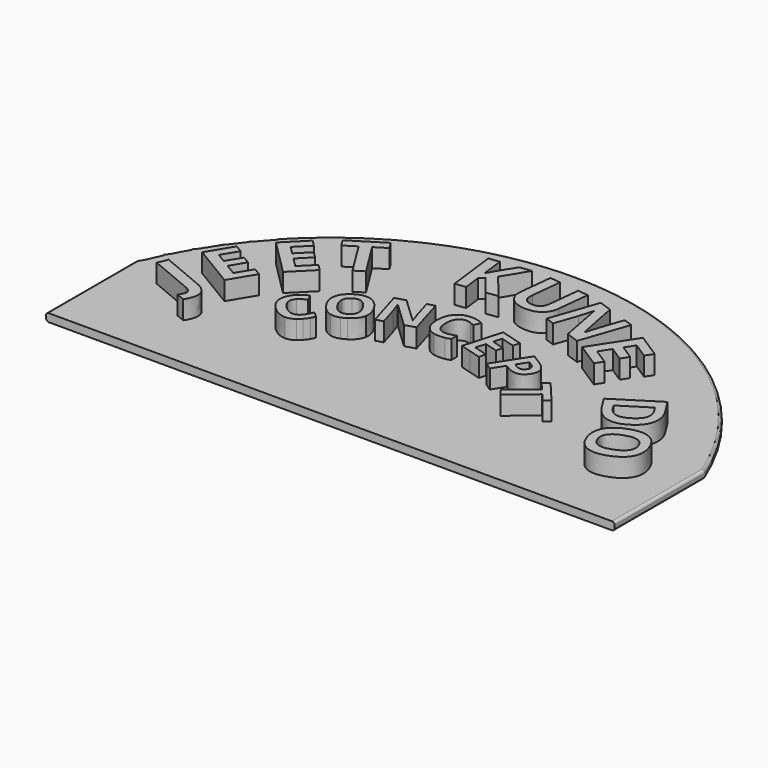
from build123d import *

# Parameters (mm, degrees)
F0_TEXT_SIZE   = 26.3888888889
F0_TEXT_SIZE_2 = 20.8333333333
F1_DEPTH       = 10
F2_W           = 106.8937070169
F2_H           = 42.4115008008
F3_DEPTH       = 3
F4_R           = 1
F5_R           = 1


# Not quite as in the source:
# - Text() gives the source's letters only with a copy of the font that has no kerning and outlines rounded to 1/6400 em; it was checked with that copy


with BuildPart() as f1:
    # F0 (on Top) → F1 (new body)
    with BuildSketch(Plane.XY):
        with BuildLine():
            add(Edge.make_bspline(
                [(-38.4091225358, 32.0256214873), (-39.979942422, 30.889467014), (-41.7688680067, 30.899920348)],
                knots=[0.3156073203, 0.3156073203, 0.3156073203, 1, 1, 1], degree=2))
            Line((-38.4091225358, 32.0256214873), (-35.6095221105, 35.256532611))
            add(Edge.make_bspline(
                [(-34.8738305014, 36.8883343337), (-35.1570391266, 36.0542519462), (-35.6095221105, 35.256532611)],
                knots=[0, 0, 0, 0.4442187703, 0.4442187703, 0.4442187703], degree=2))
            Line((-34.8738305014, 36.8883343337), (-36.8551148685, 38.6379550595))
            add(Edge.make_bspline(
                [(-38.7797452841, 35.2782195153), (-37.7433320216, 36.4518621022), (-36.8551148685, 38.6379550595)],
                knots=[0, 0, 0, 1, 1, 1], degree=2))
            add(Edge.make_bspline(
                [(-44.9795205124, 35.7719230867), (-41.2511922945, 32.4795333465), (-38.7797452841, 35.2782195153)],
                knots=[0, 0, 0, 1, 1, 1], degree=2))
            add(Edge.make_bspline(
                [(-47.1269150723, 38.9710622999), (-46.77048446, 37.3534767969), (-44.9795205124, 35.7719230867)],
                knots=[0, 0, 0, 1, 1, 1], degree=2))
            add(Edge.make_bspline(
                [(-46.3047218705, 41.9233307448), (-47.4833456845, 40.588647803), (-47.1269150723, 38.9710622999)],
                knots=[0, 0, 0, 1, 1, 1], degree=2))
            add(Edge.make_bspline(
                [(-44.9871563721, 42.9702926502), (-45.7660455386, 42.5333320894), (-46.3047218705, 41.9233307448)],
                knots=[0, 0, 0, 1, 1, 1], degree=2))
            add(Edge.make_bspline(
                [(-43.3568272803, 43.7714605433), (-44.2082672056, 43.407253211), (-44.9871563721, 42.9702926502)],
                knots=[0, 0, 0, 1, 1, 1], degree=2))
            Line((-43.3568272803, 43.7714605433), (-44.6072834562, 46.2306500193))
            add(Edge.make_bspline(
                [(-48.2713662053, 43.6600232387), (-46.8384871626, 45.2826268152), (-44.6072834562, 46.2306500193)],
                knots=[0, 0, 0, 1, 1, 1], degree=2))
            add(Edge.make_bspline(
                [(-50.0289540377, 40.2656887419), (-49.6783887841, 42.0666997267), (-48.2713662053, 43.6600232387)],
                knots=[0, 0, 0, 1, 1, 1], degree=2))
            add(Edge.make_bspline(
                [(-49.630822441, 36.6765743061), (-50.3795192913, 38.4646777572), (-50.0289540377, 40.2656887419)],
                knots=[0, 0, 0, 1, 1, 1], degree=2))
            add(Edge.make_bspline(
                [(-47.1424017561, 33.3521659566), (-48.8821255907, 34.888470855), (-49.630822441, 36.6765743061)],
                knots=[0, 0, 0, 1, 1, 1], degree=2))
            add(Edge.make_bspline(
                [(-41.7688680067, 30.899920348), (-44.3827556733, 30.9151942313), (-47.1424017561, 33.3521659566)],
                knots=[0, 0, 0, 1, 1, 1], degree=2))
        make_face()
        with BuildLine():
            Line((-35.6095221105, 35.256532611), (-38.4091225358, 32.0256214873))
            add(Edge.make_bspline(
                [(-37.0067391286, 33.3173318267), (-37.6847397807, 32.5495585185), (-38.4091225358, 32.0256214873)],
                knots=[0, 0, 0, 0.3156073203, 0.3156073203, 0.3156073203], degree=2))
            add(Edge.make_bspline(
                [(-35.6095221105, 35.256532611), (-36.1756430537, 34.2584716043), (-37.0067391286, 33.3173318267)],
                knots=[0.4442187703, 0.4442187703, 0.4442187703, 1, 1, 1], degree=2))
        make_face()
        Polygon((36.4704009429, 34.3043494452), (37.7874787177, 32.7430366973), (38.5155209345, 31.9028311896), (47.867163069, 39.7916030132), (50.4698346878, 36.7062997345), (52.4752818189, 38.3980362866), (45.2339777183, 46.9821462153), (43.2285305872, 45.2904096631), (45.8333011347, 42.2026182366), align=None)
        Polygon((38.5155209345, 31.9028311896), (37.7874787177, 32.7430366973), (38.5042628772, 31.8933342217), align=None)
        Polygon((14.3201833544, 63.3800999888), (10.2276517863, 49.1077462863), (14.0866278421, 47.9746486807), (18.4532967766, 46.7225265126), (19.1711023907, 49.2258121791), (13.9705264185, 50.7170533424), (15.0274951853, 54.4031414864), (19.8682238429, 53.0150848801), (20.5806459149, 55.4995959041), (15.7399172573, 56.8876525104), (16.639866046, 60.0261469147), (21.8404420181, 58.5349057514), (22.5528640902, 61.0194167754), align=None)
        Polygon((14.0866278421, 47.9746486807), (10.2276517863, 49.1077462863), (10.2206160409, 49.083209726), align=None)
        with BuildLine():
            add(Edge.make_bspline(
                [(-0.9883344196, 50), (-2.852809563, 50.430438258), (-4.0169270833, 51.7643229167)],
                knots=[0.3226952609, 0.3226952609, 0.3226952609, 1, 1, 1], degree=2))
            Line((-0.9883344196, 50), (3.1714734134, 50))
            add(Edge.make_bspline(
                [(5.0358072917, 50.5598958333), (4.1536014918, 50.191001949), (3.1714734134, 50)],
                knots=[0, 0, 0, 0.4822306436, 0.4822306436, 0.4822306436], degree=2))
            Line((5.0358072917, 50.5598958333), (5.0358072917, 53.203125))
            add(Edge.make_bspline(
                [(1.2434895833, 52.421875), (2.8092447917, 52.421875), (5.0358072917, 53.203125)],
                knots=[0, 0, 0, 1, 1, 1], degree=2))
            add(Edge.make_bspline(
                [(-2.490234375, 57.3958333333), (-2.490234375, 52.421875), (1.2434895833, 52.421875)],
                knots=[0, 0, 0, 1, 1, 1], degree=2))
            add(Edge.make_bspline(
                [(-1.513671875, 61.123046875), (-2.490234375, 59.78515625), (-2.490234375, 57.3958333333)],
                knots=[0, 0, 0, 1, 1, 1], degree=2))
            add(Edge.make_bspline(
                [(1.2434895833, 62.4609375), (-0.537109375, 62.4609375), (-1.513671875, 61.123046875)],
                knots=[0, 0, 0, 1, 1, 1], degree=2))
            add(Edge.make_bspline(
                [(2.900390625, 62.1663411458), (2.0572916667, 62.4609375), (1.2434895833, 62.4609375)],
                knots=[0, 0, 0, 1, 1, 1], degree=2))
            add(Edge.make_bspline(
                [(4.580078125, 61.474609375), (3.7434895833, 61.8717447917), (2.900390625, 62.1663411458)],
                knots=[0, 0, 0, 1, 1, 1], degree=2))
            Line((4.580078125, 61.474609375), (5.595703125, 64.0397135417))
            add(Edge.make_bspline(
                [(1.2434895833, 65.0846354167), (3.408203125, 65.0846354167), (5.595703125, 64.0397135417)],
                knots=[0, 0, 0, 1, 1, 1], degree=2))
            add(Edge.make_bspline(
                [(-2.4641927083, 64.1552734375), (-0.8821614583, 65.0846354167), (1.2434895833, 65.0846354167)],
                knots=[0, 0, 0, 1, 1, 1], degree=2))
            add(Edge.make_bspline(
                [(-4.8909505208, 61.4811197917), (-4.0462239583, 63.2259114583), (-2.4641927083, 64.1552734375)],
                knots=[0, 0, 0, 1, 1, 1], degree=2))
            add(Edge.make_bspline(
                [(-5.7356770833, 57.4153645833), (-5.7356770833, 59.736328125), (-4.8909505208, 61.4811197917)],
                knots=[0, 0, 0, 1, 1, 1], degree=2))
            add(Edge.make_bspline(
                [(-4.0169270833, 51.7643229167), (-5.7356770833, 53.7337239583), (-5.7356770833, 57.4153645833)],
                knots=[0, 0, 0, 1, 1, 1], degree=2))
        make_face()
        with BuildLine():
            Line((3.1714734134, 50), (-0.9883344196, 50))
            add(Edge.make_bspline(
                [(0.947265625, 49.794921875), (-0.1000233565, 49.794921875), (-0.9883344196, 50)],
                knots=[0, 0, 0, 0.3226952609, 0.3226952609, 0.3226952609], degree=2))
            add(Edge.make_bspline(
                [(3.1714734134, 50), (2.1169659288, 49.794921875), (0.947265625, 49.794921875)],
                knots=[0.4822306436, 0.4822306436, 0.4822306436, 1, 1, 1], degree=2))
        make_face()
        with BuildLine():
            Line((-24.4078682127, 60.4176286142), (-20.1662794221, 46.189501909))
            Line((-20.1662794221, 46.189501909), (-17.4614357189, 46.9837156795))
            Line((-17.4614357189, 46.9837156795), (-19.4567369945, 53.6768207319))
            add(Edge.make_bspline(
                [(-20.8584569239, 57.69514098), (-19.8203572799, 54.8965607274), (-19.4567369945, 53.6768207319)],
                knots=[0, 0, 0, 1, 1, 1], degree=2))
            Line((-20.8584569239, 57.69514098), (-20.7711098142, 57.7211802843))
            Line((-20.7711098142, 57.7211802843), (-11.3554708956, 48.7888419283))
            Line((-11.3554708956, 48.7888419283), (-7.5153176106, 49.9336413433))
            Line((-7.5153176106, 49.9336413433), (-11.7643740906, 64.1868179147))
            Line((-11.7643740906, 64.1868179147), (-14.4846126484, 63.3758795801))
            Line((-14.4846126484, 63.3758795801), (-12.4730763896, 56.6283153595))
            add(Edge.make_bspline(
                [(-11.1556193077, 52.7445237971), (-12.1308455328, 55.4803247755), (-12.4730763896, 56.6283153595)],
                knots=[0, 0, 0, 1, 1, 1], degree=2))
            Line((-11.1556193077, 52.7445237971), (-11.2242491796, 52.7240643437))
            Line((-11.2242491796, 52.7240643437), (-20.5957907844, 61.5540582528))
            Line((-20.5957907844, 61.5540582528), (-24.4078682127, 60.4176286142))
        make_face()
        Polygon((-17.4614357189, 46.9837156795), (-20.1662794221, 46.189501909), (-20.1588117327, 46.1644520429), (-17.4572904127, 46.9698105265), align=None)
        with BuildLine():
            add(Edge.make_bspline(
                [(-28.8562814175, 40.8903084305), (-30.71235981, 40.2057235951), (-32.459128248, 40.6472849951)],
                knots=[0.3326622041, 0.3326622041, 0.3326622041, 1, 1, 1], degree=2))
            Line((-28.8562814175, 40.8903084305), (-25.4297026695, 43.092436877))
            add(Edge.make_bspline(
                [(-23.6657186248, 46.3818238072), (-23.9755686621, 44.5486220381), (-25.4297026695, 43.092436877)],
                knots=[0, 0, 0, 0.6886308448, 0.6886308448, 0.6886308448], degree=2))
            add(Edge.make_bspline(
                [(-25.2339698014, 52.1386551776), (-23.2157677699, 49.0439203179), (-23.6657186248, 46.3818238072)],
                knots=[0, 0, 0, 1, 1, 1], degree=2))
            add(Edge.make_bspline(
                [(-29.8556414258, 55.9003410756), (-27.2557281361, 55.2388433145), (-25.2339698014, 52.1386551776)],
                knots=[0, 0, 0, 1, 1, 1], degree=2))
            add(Edge.make_bspline(
                [(-35.3267052065, 54.6894452338), (-32.4555547155, 56.5618388366), (-29.8556414258, 55.9003410756)],
                knots=[0, 0, 0, 1, 1, 1], degree=2))
            add(Edge.make_bspline(
                [(-38.6661217228, 50.174101002), (-38.1978556974, 52.8170516309), (-35.3267052065, 54.6894452338)],
                knots=[0, 0, 0, 1, 1, 1], degree=2))
            add(Edge.make_bspline(
                [(-37.1055168073, 44.4200556815), (-39.1343877483, 47.531150373), (-38.6661217228, 50.174101002)],
                knots=[0, 0, 0, 1, 1, 1], degree=2))
            add(Edge.make_bspline(
                [(-32.459128248, 40.6472849951), (-35.0766458663, 41.30896099), (-37.1055168073, 44.4200556815)],
                knots=[0, 0, 0, 1, 1, 1], degree=2))
        make_face()
        with BuildLine():
            add(Edge.make_bspline(
                [(-34.3245830367, 46.2102978444), (-32.9625189344, 44.121692644), (-31.4813966754, 43.5816732008)],
                knots=[0, 0, 0, 1, 1, 1], degree=2))
            add(Edge.make_bspline(
                [(-35.5763015064, 49.878726324), (-35.6848689875, 48.2961764062), (-34.3245830367, 46.2102978444)],
                knots=[0, 0, 0, 1, 1, 1], degree=2))
            add(Edge.make_bspline(
                [(-33.8917368898, 52.489047849), (-35.4677340253, 51.4612762417), (-35.5763015064, 49.878726324)],
                knots=[0, 0, 0, 1, 1, 1], degree=2))
            add(Edge.make_bspline(
                [(-28.0042346626, 50.3320531828), (-30.7479225345, 54.5392566088), (-33.8917368898, 52.489047849)],
                knots=[0, 0, 0, 1, 1, 1], degree=2))
            add(Edge.make_bspline(
                [(-28.4242772808, 44.069425365), (-25.2641030937, 46.1303030342), (-28.0042346626, 50.3320531828)],
                knots=[0, 0, 0, 1, 1, 1], degree=2))
            add(Edge.make_bspline(
                [(-31.4813966754, 43.5816732008), (-30.0002744164, 43.0416537577), (-28.4242772808, 44.069425365)],
                knots=[0, 0, 0, 1, 1, 1], degree=2))
        make_face(mode=Mode.SUBTRACT)
        with BuildLine():
            Line((-25.4297026695, 43.092436877), (-28.8562814175, 40.8903084305))
            add(Edge.make_bspline(
                [(-26.9786400547, 41.8526681483), (-27.9310421565, 41.2315681369), (-28.8562814175, 40.8903084305)],
                knots=[0, 0, 0, 0.3326622041, 0.3326622041, 0.3326622041], degree=2))
            add(Edge.make_bspline(
                [(-25.4297026695, 43.092436877), (-26.0871993253, 42.434012778), (-26.9786400547, 41.8526681483)],
                knots=[0.6886308448, 0.6886308448, 0.6886308448, 1, 1, 1], degree=2))
        make_face()
        with Locations(Location((-76.3449299567, 24.9456217643), (0, 0, 67.29))):
            Text('J', F0_TEXT_SIZE, font='Open Sans', font_style=FontStyle.BOLD, text_align=(TextAlign.LEFT, TextAlign.BOTTOM))
        with Locations(Location((-71.5827823484, 36.1636671281), (0, 0, 59))):
            Text('E', F0_TEXT_SIZE, font='Open Sans', font_style=FontStyle.BOLD, text_align=(TextAlign.LEFT, TextAlign.BOTTOM))
        with Locations(Location((-61.847214309, 51.2898706808), (0, 0, 45))):
            Text('E', F0_TEXT_SIZE, font='Open Sans', font_style=FontStyle.BOLD, text_align=(TextAlign.LEFT, TextAlign.BOTTOM))
        with Locations(Location((-49.5437797618, 63.3755894952), (0, 0, 32))):
            Text('T', F0_TEXT_SIZE, font='Open Sans', font_style=FontStyle.BOLD, text_align=(TextAlign.LEFT, TextAlign.BOTTOM))
        with Locations(Location((-18.5029836255, 78.3248967944), (0, 0, 7))):
            Text('K', F0_TEXT_SIZE, font='Open Sans', font_style=FontStyle.BOLD, text_align=(TextAlign.LEFT, TextAlign.BOTTOM))
        with Locations(Location((-0.6942829813, 80.5454588178), (0, 0, -6.2))):
            Text('U', F0_TEXT_SIZE, font='Open Sans', font_style=FontStyle.BOLD, text_align=(TextAlign.LEFT, TextAlign.BOTTOM))
        with Locations(Location((16.5919480729, 78.8955366347), (0, 0, -19))):
            Text('N', F0_TEXT_SIZE, font='Open Sans', font_style=FontStyle.BOLD, text_align=(TextAlign.LEFT, TextAlign.BOTTOM))
        with Locations(Location((36.301748369, 71.8037585262), (0, 0, -33))):
            Text('E', F0_TEXT_SIZE, font='Open Sans', font_style=FontStyle.BOLD, text_align=(TextAlign.LEFT, TextAlign.BOTTOM))
        with Locations(Location((62.4652452618, 50.8903824765), (0, 0, -57.6603795557))):
            Text('D', F0_TEXT_SIZE, font='Open Sans', font_style=FontStyle.BOLD, text_align=(TextAlign.LEFT, TextAlign.BOTTOM))
        with Locations(Location((21.3617728091, 45.7211184839), (0, 0, -32.83))):
            Text('P', F0_TEXT_SIZE_2, font='Open Sans', font_style=FontStyle.BOLD, text_align=(TextAlign.LEFT, TextAlign.BOTTOM))
        with Locations(Location((71.8190781505, 36.3487066861), (0, 0, -69.6))):
            Text('O', F0_TEXT_SIZE, font='Open Sans', font_style=FontStyle.BOLD, text_align=(TextAlign.LEFT, TextAlign.BOTTOM))
    extrude(amount=F1_DEPTH)

    # F2 (on Top) → F3 (join)
    with BuildSketch(Plane.XY):
        with BuildLine():
            Line((0, 42.4115008008), (106.8937070169, 42.4115008008))
            ThreePointArc((106.8937070169, 42.4115008008), (0, 115), (-106.8937070169, 42.4115008008))
            Line((-106.8937070169, 42.4115008008), (-106.8937070169, 0))
            Line((-106.8937070169, 0), (0, 0))
            Line((0, 0), (0, 42.4115008008))
        make_face()
        with Locations((53.4468535085, 21.2057504004)):
            Rectangle(F2_W, F2_H)
    extrude(amount=F3_DEPTH)

    # F4
    f4_edges = [f1.edges().sort_by_distance(p)[0] for p in [
        (0, 115, 3),
        (-106.893707, 21.20575, 3),
        (106.893707, 21.20575, 3),
    ]]
    fillet(f4_edges, radius=F4_R)

    # F5
    f5_edges = [f1.edges().sort_by_distance(p)[0] for p in [
        (0, 115, 0),
        (-106.893707, 21.20575, 0),
        (106.893707, 21.20575, 0),
    ]]
    fillet(f5_edges, radius=F5_R)


solid = f1.part
